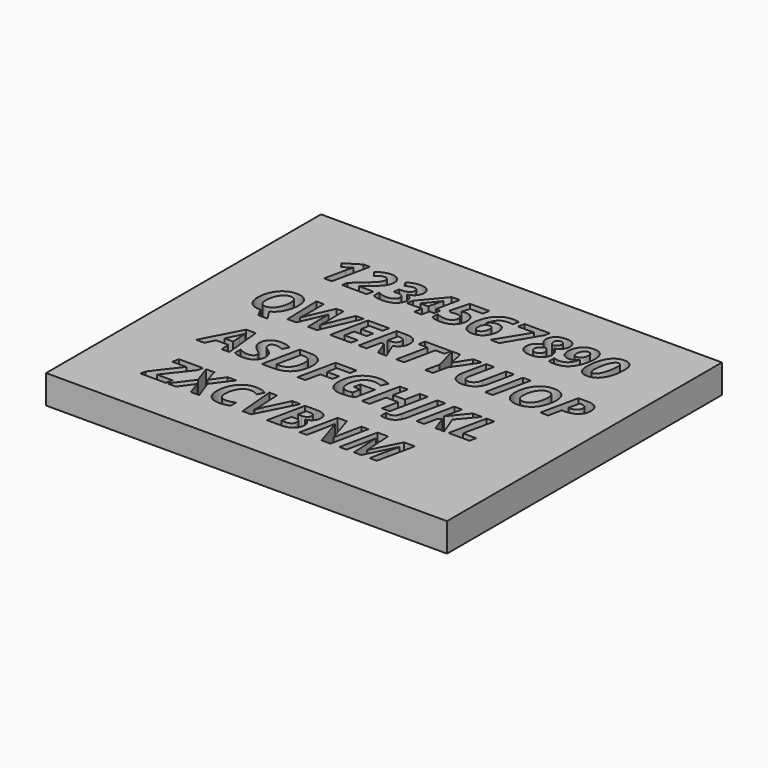
from build123d import *

# Parameters (mm, degrees)
F0_TEXT_SIZE = 46.0255058011
F1_DEPTH     = 25
F2_W         = 350
F2_H         = 300
F3_DEPTH     = 25


# Not quite as in the source:
# - Text() gives the source's letters only with a copy of the font that has no kerning and outlines rounded to 1/6400 em; it was checked with that copy


with BuildPart() as f1:
    # F0 (on Top) → F1 (new body)
    with BuildSketch(Plane.XY):
        with Locations((-2.2064675156, -16.1247980784)):
            Text('1234567890', F0_TEXT_SIZE, font='Open Sans', font_style=FontStyle.BOLDITALIC, text_align=(TextAlign.LEFT, TextAlign.BOTTOM))
        with Locations((-14.1659075386, -78.719485968)):
            Text('QWERTYUIOP', F0_TEXT_SIZE, font='Open Sans', font_style=FontStyle.BOLDITALIC, text_align=(TextAlign.LEFT, TextAlign.BOTTOM))
        with Locations((-2.2064675156, -141.3141738575)):
            Text('ASDFGHJKL', F0_TEXT_SIZE, font='Open Sans', font_style=FontStyle.BOLDITALIC, text_align=(TextAlign.LEFT, TextAlign.BOTTOM))
        with Locations((-2.2064675156, -203.9088617471)):
            Text('ZXCVBNM', F0_TEXT_SIZE, font='Open Sans', font_style=FontStyle.BOLDITALIC, text_align=(TextAlign.LEFT, TextAlign.BOTTOM))
    extrude(amount=F1_DEPTH)


with BuildPart() as f3:
    # F2 (on Top) → F3 (new body)
    with BuildSketch(Plane.XY):
        with Locations((120.7755804062, -93.5788617471)):
            Rectangle(F2_W, F2_H)
    extrude(amount=F3_DEPTH)

    # F4: cut F1
    add(f1.part, mode=Mode.SUBTRACT)


solid = f3.part
